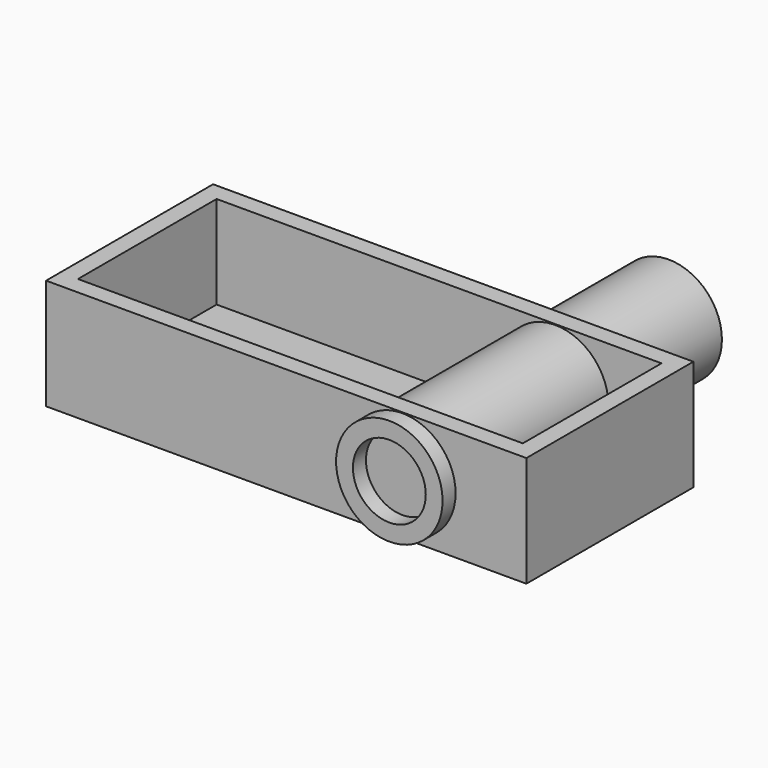
from build123d import *

# Parameters (mm, degrees)
F0_W          = 108.5266880691
F0_H          = 47.1645910293
F1_DEPTH      = 25
F2_T          = -4
F3_R          = 12.0317315012
F3_R_2        = 8.2327991294
F4_DEPTH      = 30
F4_DEPTH_BACK = 30
F5_DEPTH      = 78.9


with BuildPart() as f1:
    # F0 (on Top) → F1 (new body)
    with BuildSketch(Plane.XY):
        with Locations((10.1203862578, -2.7356250212)):
            Rectangle(F0_W, F0_H)
    extrude(amount=F1_DEPTH)

    # F2
    f2_openings = [f1.faces().sort_by_distance(p)[0] for p in [
        (10.120386, -2.735625, 25),
    ]]
    offset(amount=F2_T, openings=f2_openings)


with BuildPart() as f4:
    # F3 (on Front) → F4 (new body, two sides)
    with BuildSketch(Plane.XZ) as f4_sk:
        with Locations((36.3620221615, 12.7822495997)):
            Circle(F3_R)
        with Locations((36.3620221615, 12.7822495997)):
            Circle(F3_R_2, mode=Mode.SUBTRACT)
    extrude(amount=F4_DEPTH)
    extrude(f4_sk.sketch, amount=-F4_DEPTH_BACK)

    # F5 (add): a face of the model
    f5_faces = [f4.faces().sort_by_distance(p)[0] for p in [
        (24.6705994176, -30, 12.7822495997),
    ]]
    extrude(f5_faces, amount=-F5_DEPTH)


solid = Compound([f1.part, f4.part])
